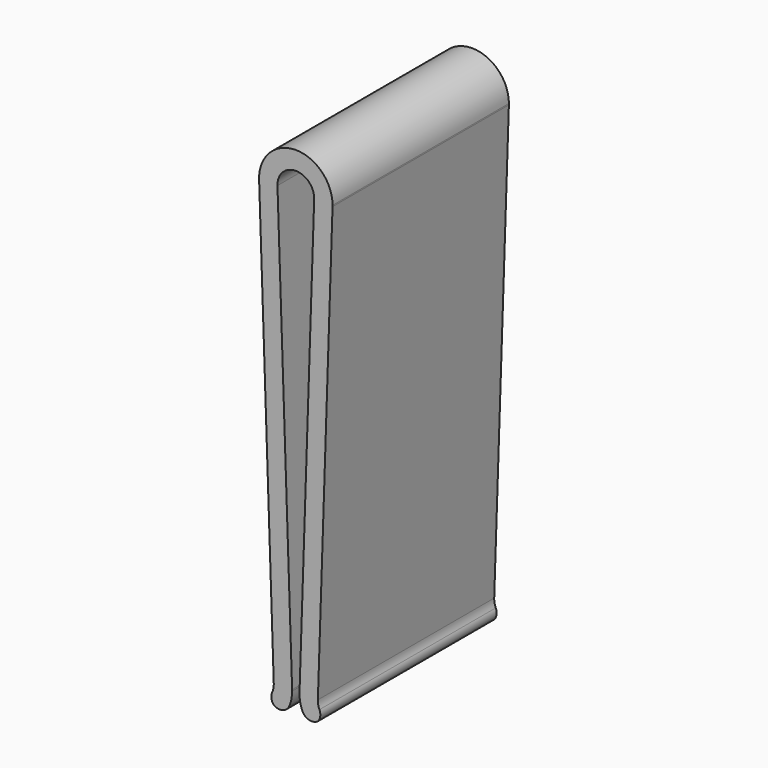
from build123d import *

# Parameters (mm, degrees)
F1_DEPTH    = 19.05
F2_T1_DEPTH = 22.6696744492
F2_T3_DEPTH = 25.3488085544


# Not quite as in the source:
# - a fillet or chamfer that OpenCascade refuses, or shapes differently, is made with other operations: its cross-section is extruded or revolved along the edge and cut away or added


with BuildPart() as f1:
    # F0 (on Front) → F1 (new body)
    with BuildSketch(Plane.XZ):
        with BuildLine():
            ThreePointArc((-1.586615103, -0.0529977822), (-0.0265025846, 1.5872787603), (1.5875, 0))
            ThreePointArc((1.5875, 0), (1.5872787603, -0.0265025846), (1.586615103, -0.0529977822))
            Line((1.586615103, -0.0529977822), (1.4948202515, -2.8010957527))
            ThreePointArc((1.4948202515, -2.8010957527), (2.6951001882, -1.6784099545), (3.173230206, -0.1059955644))
            ThreePointArc((3.173230206, -0.1059955644), (3.1745575207, -0.0530051692), (3.175, 0))
            ThreePointArc((3.175, 0), (-0.0530051692, 3.1745575207), (-3.173230206, -0.1059955644))
            ThreePointArc((-3.173230206, -0.1059955644), (-2.6951001882, -1.6784099545), (-1.4948202515, -2.8010957527))
            Line((-1.4948202515, -2.8010957527), (-1.586615103, -0.0529977822))
        make_face()
        with BuildLine():
            Line((-0.319269794, -37.9940044356), (-1.4948202515, -2.8010957527))
            ThreePointArc((-1.4948202515, -2.8010957527), (-2.6951001882, -1.6784099545), (-3.173230206, -0.1059955644))
            Line((-3.173230206, -0.1059955644), (-1.9976797485, -35.2989042473))
            ThreePointArc((-1.9976797485, -35.2989042473), (-0.7973998118, -36.4215900455), (-0.319269794, -37.9940044356))
        make_face()
        with BuildLine():
            ThreePointArc((3.173230206, -0.1059955644), (2.6951001882, -1.6784099545), (1.4948202515, -2.8010957527))
            Line((1.4948202515, -2.8010957527), (0.319269794, -37.9940044356))
            ThreePointArc((0.319269794, -37.9940044356), (0.7973998118, -36.4215900455), (1.9976797485, -35.2989042473))
            Line((1.9976797485, -35.2989042473), (3.173230206, -0.1059955644))
        make_face()
        with BuildLine():
            ThreePointArc((-0.3175, -38.1), (-0.3179424793, -38.0469948308), (-0.319269794, -37.9940044356))
            ThreePointArc((-0.319269794, -37.9940044356), (-0.7973998118, -36.4215900455), (-1.9976797485, -35.2989042473))
            Line((-1.9976797485, -35.2989042473), (-1.905884897, -38.0470022178))
            ThreePointArc((-1.905884897, -38.0470022178), (-1.9052212397, -38.0734974154), (-1.905, -38.1))
            ThreePointArc((-1.905, -38.1), (-2.0258412421, -38.7075099489), (-2.3699679849, -39.2225320151))
            Line((-2.3699679849, -39.2225320151), (-1.2474359697, -40.3450640303))
            ThreePointArc((-1.2474359697, -40.3450640303), (-0.5591824843, -39.3150198978), (-0.3175, -38.1))
        make_face()
        with BuildLine():
            ThreePointArc((1.9976797485, -35.2989042473), (0.7973998118, -36.4215900455), (0.319269794, -37.9940044356))
            ThreePointArc((0.319269794, -37.9940044356), (0.5393070818, -39.2658801773), (1.2474359697, -40.3450640303))
            Line((1.2474359697, -40.3450640303), (2.3699679849, -39.2225320151))
            ThreePointArc((2.3699679849, -39.2225320151), (2.0159035409, -38.6829400886), (1.905884897, -38.0470022178))
            Line((1.905884897, -38.0470022178), (1.9976797485, -35.2989042473))
        make_face()
    extrude(amount=F1_DEPTH)

    # F2: fillet of radius 0.889 on 4 edges, made by hand

    # F2_s2 → F2_t1 (cut)
    with BuildSketch(Plane.XZ.offset(-1.8098372246)):
        with BuildLine():
            ThreePointArc((-2.0418274273, -38.7447521515), (-2.1035117306, -39.2681046567), (-1.8580687151, -39.7344312849))
            Line((-1.8580687151, -39.7344312849), (-2.3699679849, -39.2225320151))
            ThreePointArc((-2.3699679849, -39.2225320151), (-2.1839076792, -38.9987448959), (-2.0418274273, -38.7447521515))
        make_face()
        with BuildLine():
            ThreePointArc((1.8580687151, -39.7344312849), (2.1035117306, -39.2681046567), (2.0418274273, -38.7447521515))
            ThreePointArc((2.0418274273, -38.7447521515), (2.1839076792, -38.9987448959), (2.3699679849, -39.2225320151))
            Line((2.3699679849, -39.2225320151), (1.8580687151, -39.7344312849))
        make_face()
    extrude(amount=F2_T1_DEPTH, mode=Mode.SUBTRACT)

    # F2_s4 → F2_t3 (cut)
    with BuildSketch(Plane.XZ.offset(-3.1494042772)):
        with BuildLine():
            ThreePointArc((-2.0032929963, -39.5892070037), (-1.1983084283, -39.8319189832), (-0.551076483, -39.2952626045))
            ThreePointArc((-0.551076483, -39.2952626045), (-0.8466666667, -39.8550472849), (-1.2474359697, -40.3450640303))
            Line((-1.2474359697, -40.3450640303), (-2.0032929963, -39.5892070037))
        make_face()
        with BuildLine():
            ThreePointArc((0.551076483, -39.2952626045), (1.1983084283, -39.8319189832), (2.0032929963, -39.5892070037))
            Line((2.0032929963, -39.5892070037), (1.2474359697, -40.3450640303))
            ThreePointArc((1.2474359697, -40.3450640303), (0.8466666667, -39.8550472849), (0.551076483, -39.2952626045))
        make_face()
    extrude(amount=F2_T3_DEPTH, mode=Mode.SUBTRACT)


solid = f1.part
